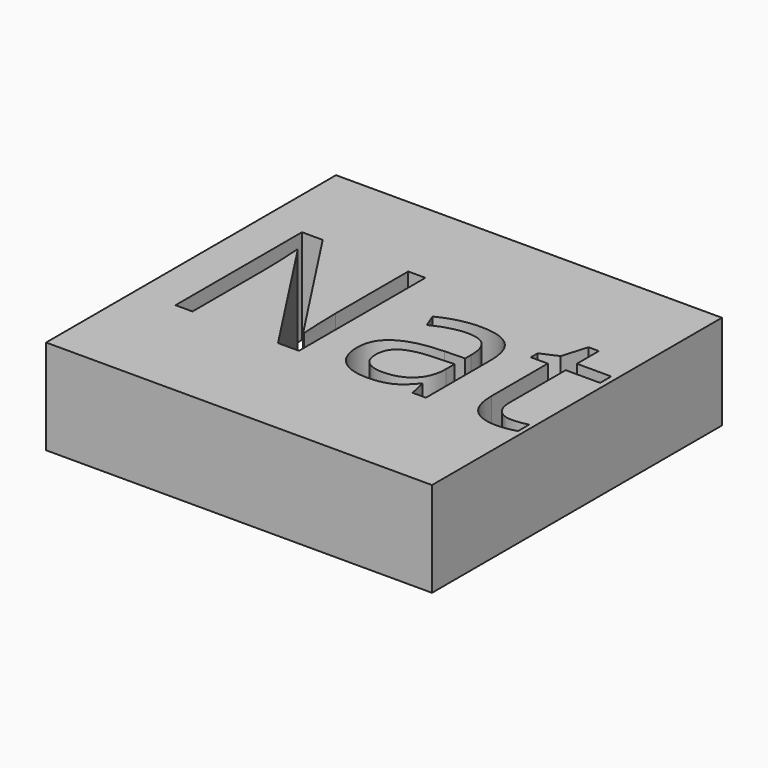
from build123d import *

# Parameters (mm, degrees)
F0_W         = 162.1889397502
F0_H         = 152.3081883788
F1_DEPTH     = 39.878
F2_TEXT_SIZE = 93.0504562954
F3_DEPTH     = 80.518


# Not quite as in the source:
# - Text() gives the source's letters only with a copy of the font that has no kerning and outlines rounded to 1/6400 em; it was checked with that copy


with BuildPart() as f1:
    # F0 (on Top) → F1 (new body)
    with BuildSketch(Plane.XY):
        with Locations((-1.4459677041, -2.2894404829)):
            Rectangle(F0_W, F0_H)
    extrude(amount=F1_DEPTH)

    # F2 (on face) → F3 (cut)
    with BuildSketch(Plane.XY.offset(39.878)):
        with Locations((-75.0696212053, -31.2087200582)):
            Text('Natneut', F2_TEXT_SIZE, font='Open Sans', text_align=(TextAlign.LEFT, TextAlign.BOTTOM))
    extrude(amount=-F3_DEPTH, mode=Mode.SUBTRACT)


solid = f1.part
